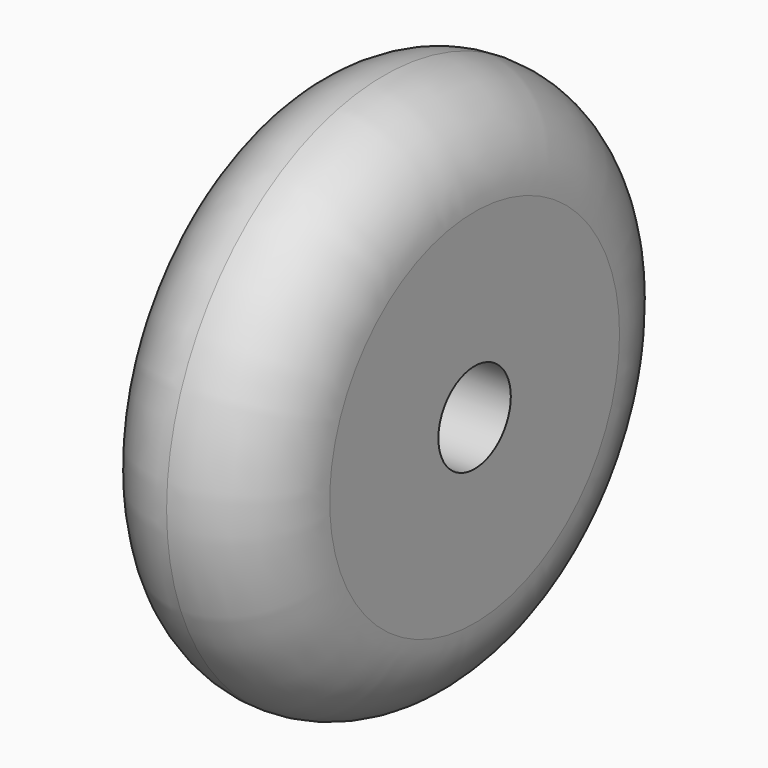
from build123d import *

# Parameters (mm, degrees)
F0_R     = 9.525
F0_R_2   = 1.5875
F1_DEPTH = 6.35
F2_R     = 3.17499


# Not quite as in the source:
# - a fillet or chamfer is up to 0.001 mm smaller than in the source, because OpenCascade refuses the exact size


with BuildPart() as f1:
    # F0 (on Right) → F1 (new body)
    with BuildSketch(Plane.YZ):
        Circle(F0_R)
        Circle(F0_R_2, mode=Mode.SUBTRACT)
    extrude(amount=F1_DEPTH)

    # F2 (radius 3.175 in the source; OpenCascade refuses exactly that, so slightly less here)
    f2_edges = [f1.edges().sort_by_distance(p)[0] for p in [
        (6.35, -9.525, 0),
        (0, -9.525, 0),
    ]]
    fillet(f2_edges, radius=F2_R)


solid = f1.part
